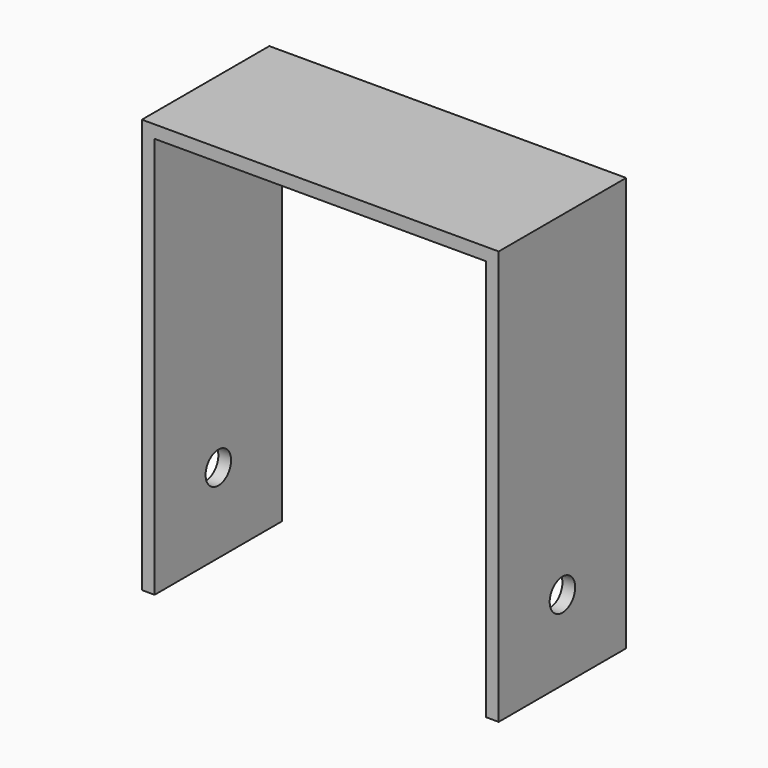
from build123d import *

# Parameters (mm, degrees)
F1_DEPTH      = 12.5
F2_R          = 2.5
F3_DEPTH      = 56.001
F3_DEPTH_BACK = 126


# Not quite as in the source:
# - an extrude ends at something that could not be found from the text; its depth is read off the source's solid


with BuildPart() as f1:
    # F0 (on Front) → F1 (new body, symmetric)
    with BuildSketch(Plane.XZ):
        Polygon((-2, -65), (0, -65), (0, 0), (-56, 0), (-56, -65), (-54, -65), (-54, -2), (-2, -2), align=None)
    extrude(amount=F1_DEPTH, both=True)

    # F2 (on Right) → F3 (cut, two sides)
    with BuildSketch(Plane.YZ) as f3_sk:
        with Locations((0, -52.5)):
            Circle(F2_R)
    extrude(amount=-F3_DEPTH, mode=Mode.SUBTRACT)
    extrude(f3_sk.sketch, amount=F3_DEPTH_BACK, mode=Mode.SUBTRACT)


solid = f1.part
